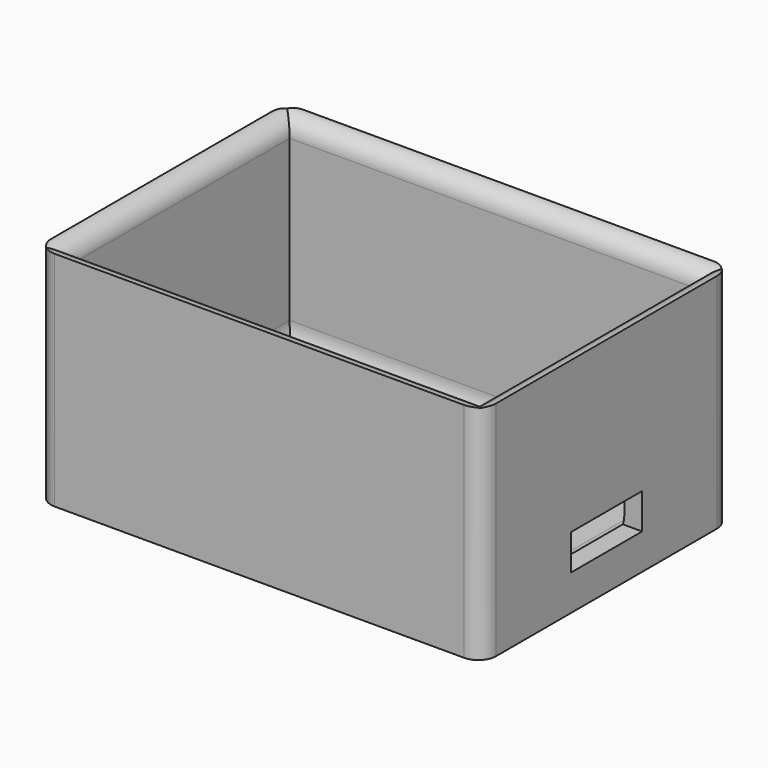
from build123d import *

# Parameters (mm, degrees)
F1_DEPTH     = 25
F2_T         = 2
F3_T1_DEPTH  = 31
F3_T3_DEPTH  = 46
F3_T9_DEPTH  = 51
F3_T13_DEPTH = 36
F3_T20_DEPTH = 36
F3_T24_DEPTH = 51
F3_T31_DEPTH = 36
F3_T35_DEPTH = 51
F3_T42_DEPTH = 36
F3_T46_DEPTH = 51
F4_R         = 3
F5_R         = 1
F6_DEPTH     = 4
F8_W         = 10
F8_H         = 4
F9_DEPTH     = 4


# Not quite as in the source:
# - a fillet or chamfer that OpenCascade refuses, or shapes differently, is made with other operations: its cross-section is extruded or revolved along the edge and cut away or added
# - a shell that OpenCascade refuses in one call is made with other operations: the cavity is built on its own and cut out


with BuildPart() as f1:
    # F0 (on Top) → F1 (new body)
    with BuildSketch(Plane.XY):
        with BuildLine():
            ThreePointArc((25, 15.5), (24.4142135624, 16.9142135624), (23, 17.5))
            Line((23, 17.5), (-23, 17.5))
            ThreePointArc((-23, 17.5), (-24.4142135624, 16.9142135624), (-25, 15.5))
            Line((-25, 15.5), (-25, -15.5))
            ThreePointArc((-25, -15.5), (-24.4142135624, -16.9142135624), (-23, -17.5))
            Line((-23, -17.5), (23, -17.5))
            ThreePointArc((23, -17.5), (24.4142135624, -16.9142135624), (25, -15.5))
            Line((25, -15.5), (25, 15.5))
        make_face()
    extrude(amount=F1_DEPTH)

    # F2: shell of thickness 2, made by hand


with BuildPart() as f2_core1:
    # F2_t2: copy of F1
    add(f1.part)

    # the walls: a layer under each face that stays
    f2_faces = [f2_core1.faces().sort_by_distance(p)[0] for p in [
        (0, 17.5, 12.5),
        (-25, 0, 12.5),
        (0, -17.5, 12.5),
        (25, 0, 12.5),
        (0, 0, 0),
    ]]
    thicken(f2_faces, amount=-F2_T, mode=Mode.SUBTRACT)


with BuildPart() as f1_1:
    add(f1.part)

    # what is left inside the walls is the cavity
    f2_cavity = [f2_core1.part.solids().sort_by_distance(p)[0] for p in [
        (0, -5.166667, 2.02),
    ]]
    add(f2_cavity, mode=Mode.SUBTRACT)

    # F3: fillet of radius 2 on 4 edges, made by hand

    # F3_s2 → F3_t1 (cut)
    with BuildSketch(Plane.XZ.offset(-15.5)):
        with BuildLine():
            ThreePointArc((-25, 25), (-23.5857864376, 24.4142135624), (-23, 23))
            Line((-23, 23), (-22.96, 23))
            Line((-22.96, 23), (-22.96, 25.04))
            Line((-22.96, 25.04), (-25, 25.04))
            Line((-25, 25.04), (-25, 25))
        make_face()
        with BuildLine():
            ThreePointArc((25, 25), (23.5857864376, 24.4142135624), (23, 23))
            Line((23, 23), (22.96, 23))
            Line((22.96, 23), (22.96, 25.04))
            Line((22.96, 25.04), (25, 25.04))
            Line((25, 25.04), (25, 25))
        make_face()
    extrude(amount=F3_T1_DEPTH, mode=Mode.SUBTRACT)

    # F3_s4 → F3_t3 (cut)
    with BuildSketch(Plane.YZ.offset(-23)):
        with BuildLine():
            ThreePointArc((17.5, 25), (16.0857864376, 24.4142135624), (15.5, 23))
            Line((15.5, 23), (15.46, 23))
            Line((15.46, 23), (15.46, 25.04))
            Line((15.46, 25.04), (17.5, 25.04))
            Line((17.5, 25.04), (17.5, 25))
        make_face()
        with BuildLine():
            ThreePointArc((-17.5, 25), (-16.0857864376, 24.4142135624), (-15.5, 23))
            Line((-15.5, 23), (-15.46, 23))
            Line((-15.46, 23), (-15.46, 25.04))
            Line((-15.46, 25.04), (-17.5, 25.04))
            Line((-17.5, 25.04), (-17.5, 25))
        make_face()
    extrude(amount=F3_T3_DEPTH, mode=Mode.SUBTRACT)


with BuildPart() as f3_tool7:
    # F3_s8 → F3_t9 (new body)
    with BuildSketch(Plane.YZ.offset(23)):
        with BuildLine():
            ThreePointArc((17.5, 25), (16.0857864376, 24.4142135624), (15.5, 23))
            Line((15.5, 23), (15.46, 23))
            Line((15.46, 23), (15.46, 25.04))
            Line((15.46, 25.04), (17.5, 25.04))
            Line((17.5, 25.04), (17.5, 25))
        make_face()
    extrude(amount=-F3_T9_DEPTH)

    split(bisect_by=Plane.YZ.offset(-23), keep=Keep.BOTTOM)


with BuildPart() as f3_tool11:
    # F3_s12 → F3_t13 (new body)
    with BuildSketch(Plane.XZ.offset(-20.5)):
        with BuildLine():
            ThreePointArc((-25, 25), (-23.5857864376, 24.4142135624), (-23, 23))
            Line((-23, 23), (-22.96, 23))
            Line((-22.96, 23), (-22.96, 25.04))
            Line((-22.96, 25.04), (-25, 25.04))
            Line((-25, 25.04), (-25, 25))
        make_face()
    extrude(amount=F3_T13_DEPTH)

    split(bisect_by=Plane.XZ.offset(-15.5), keep=Keep.BOTTOM)


with BuildPart() as f3_tool7_1:
    add(f3_tool7.part)

    # F3_t15: intersect F3_tool11
    add(f3_tool11.part, mode=Mode.INTERSECT)


with BuildPart() as f1_2:
    add(f1_1.part)

    # F3_t5: cut F3_tool7
    add(f3_tool7_1.part, mode=Mode.SUBTRACT)


with BuildPart() as f3_tool18:
    # F3_s19 → F3_t20 (new body)
    with BuildSketch(Plane.XZ.offset(-15.5)):
        with BuildLine():
            ThreePointArc((-25, 25), (-23.5857864376, 24.4142135624), (-23, 23))
            Line((-23, 23), (-22.96, 23))
            Line((-22.96, 23), (-22.96, 25.04))
            Line((-22.96, 25.04), (-25, 25.04))
            Line((-25, 25.04), (-25, 25))
        make_face()
    extrude(amount=F3_T20_DEPTH)

    split(bisect_by=Plane.XZ.offset(15.5), keep=Keep.TOP)


with BuildPart() as f3_tool22:
    # F3_s23 → F3_t24 (new body)
    with BuildSketch(Plane.YZ.offset(-28)):
        with BuildLine():
            ThreePointArc((-17.5, 25), (-16.0857864376, 24.4142135624), (-15.5, 23))
            Line((-15.5, 23), (-15.46, 23))
            Line((-15.46, 23), (-15.46, 25.04))
            Line((-15.46, 25.04), (-17.5, 25.04))
            Line((-17.5, 25.04), (-17.5, 25))
        make_face()
    extrude(amount=F3_T24_DEPTH)

    split(bisect_by=Plane.YZ.offset(-23), keep=Keep.BOTTOM)


with BuildPart() as f3_tool18_1:
    add(f3_tool18.part)

    # F3_t26: intersect F3_tool22
    add(f3_tool22.part, mode=Mode.INTERSECT)


with BuildPart() as f1_3:
    add(f1_2.part)

    # F3_t16: cut F3_tool18
    add(f3_tool18_1.part, mode=Mode.SUBTRACT)


with BuildPart() as f3_tool29:
    # F3_s30 → F3_t31 (new body)
    with BuildSketch(Plane.XZ.offset(15.5)):
        with BuildLine():
            ThreePointArc((25, 25), (23.5857864376, 24.4142135624), (23, 23))
            Line((23, 23), (22.96, 23))
            Line((22.96, 23), (22.96, 25.04))
            Line((22.96, 25.04), (25, 25.04))
            Line((25, 25.04), (25, 25))
        make_face()
    extrude(amount=-F3_T31_DEPTH)

    split(bisect_by=Plane.XZ.offset(-15.5), keep=Keep.BOTTOM)


with BuildPart() as f3_tool33:
    # F3_s34 → F3_t35 (new body)
    with BuildSketch(Plane.YZ.offset(28)):
        with BuildLine():
            ThreePointArc((17.5, 25), (16.0857864376, 24.4142135624), (15.5, 23))
            Line((15.5, 23), (15.46, 23))
            Line((15.46, 23), (15.46, 25.04))
            Line((15.46, 25.04), (17.5, 25.04))
            Line((17.5, 25.04), (17.5, 25))
        make_face()
    extrude(amount=-F3_T35_DEPTH)

    split(bisect_by=Plane.YZ.offset(23), keep=Keep.TOP)


with BuildPart() as f3_tool29_1:
    add(f3_tool29.part)

    # F3_t37: intersect F3_tool33
    add(f3_tool33.part, mode=Mode.INTERSECT)


with BuildPart() as f1_4:
    add(f1_3.part)

    # F3_t27: cut F3_tool29
    add(f3_tool29_1.part, mode=Mode.SUBTRACT)


with BuildPart() as f3_tool40:
    # F3_s41 → F3_t42 (new body)
    with BuildSketch(Plane.XZ.offset(20.5)):
        with BuildLine():
            ThreePointArc((25, 25), (23.5857864376, 24.4142135624), (23, 23))
            Line((23, 23), (22.96, 23))
            Line((22.96, 23), (22.96, 25.04))
            Line((22.96, 25.04), (25, 25.04))
            Line((25, 25.04), (25, 25))
        make_face()
    extrude(amount=-F3_T42_DEPTH)

    split(bisect_by=Plane.XZ.offset(15.5), keep=Keep.TOP)


with BuildPart() as f3_tool44:
    # F3_s45 → F3_t46 (new body)
    with BuildSketch(Plane.YZ.offset(-23)):
        with BuildLine():
            ThreePointArc((-17.5, 25), (-16.0857864376, 24.4142135624), (-15.5, 23))
            Line((-15.5, 23), (-15.46, 23))
            Line((-15.46, 23), (-15.46, 25.04))
            Line((-15.46, 25.04), (-17.5, 25.04))
            Line((-17.5, 25.04), (-17.5, 25))
        make_face()
    extrude(amount=F3_T46_DEPTH)

    split(bisect_by=Plane.YZ.offset(23), keep=Keep.TOP)


with BuildPart() as f3_tool40_1:
    add(f3_tool40.part)

    # F3_t48: intersect F3_tool44
    add(f3_tool44.part, mode=Mode.INTERSECT)


with BuildPart() as f1_5:
    add(f1_4.part)

    # F3_t38: cut F3_tool40
    add(f3_tool40_1.part, mode=Mode.SUBTRACT)

    # F4
    f4_edges = [f1_5.edges().sort_by_distance(p)[0] for p in [
        (0, 15.5, 2),
        (23, 0, 2),
        (0, -15.5, 2),
        (-23, 0, 2),
    ]]
    fillet(f4_edges, radius=F4_R)

    # F5 (on Top) → F6 (join)
    with BuildSketch(Plane.XY):
        with Locations((-9, 4.5)):
            Circle(F5_R)
        with Locations((-9, -5.5)):
            Circle(F5_R)
        with Locations((9, 4.5)):
            Circle(F5_R)
        with Locations((9, -5.5)):
            Circle(F5_R)
    extrude(amount=F6_DEPTH)

    # F8 (on offset) → F9 (cut, symmetric)
    with BuildSketch(Plane.YZ.offset(23.5)):
        with Locations((0, 6)):
            Rectangle(F8_W, F8_H)
    extrude(amount=F9_DEPTH, both=True, mode=Mode.SUBTRACT)


solid = f1_5.part
